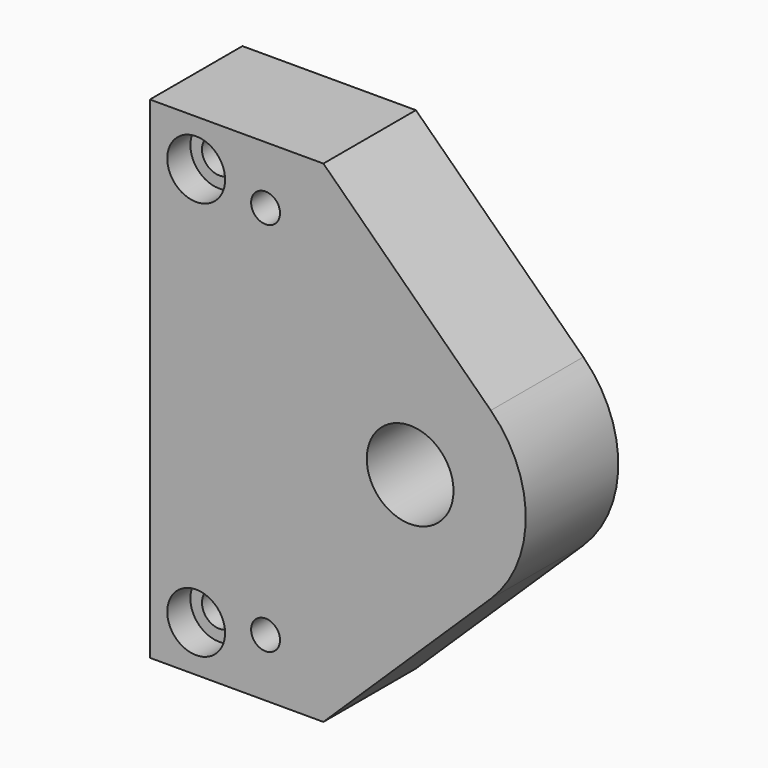
from build123d import *

# Parameters (mm, degrees)
F0_R           = 7.5
F1_DEPTH       = 20
F2_R           = 2.5
F3_DEPTH       = 20
F5_D           = 6
F5_DEPTH       = 20
F5_CBORE_D     = 10
F5_CBORE_DEPTH = 5
F5_TIP         = 1.8025818571


# Not quite as in the source:
# - a pattern or mirror of a feature is missing from the dataset's text; its kind, count and spacing are read off the source's solid


with BuildPart() as f1:
    # F0 (on Front) → F1 (new body)
    with BuildSketch(Plane.XZ):
        with BuildLine():
            Line((0, 42.5), (-30, 42.5))
            Line((-30, 42.5), (-30, -42.5))
            Line((-30, -42.5), (0, -42.5))
            Line((0, -42.5), (28.9472864716, -14.3343364017))
            ThreePointArc((28.9472864716, -14.3343364017), (35, 0), (28.9472864716, 14.3343364017))
            Line((28.9472864716, 14.3343364017), (0, 42.5))
        make_face()
        with Locations((15, 0)):
            Circle(F0_R, mode=Mode.SUBTRACT)
    extrude(amount=F1_DEPTH)

    # F2 (on face) → F3 (cut, through all)
    with BuildSketch(Plane.XZ.offset(20)):
        with Locations((-10, 32.5)):
            Circle(F2_R)
        with Locations((-10, -32.5)):
            Circle(F2_R)
    extrude(amount=-F3_DEPTH, mode=Mode.SUBTRACT)

    # F5
    with Locations(Plane.XZ.offset(20)):
        with Locations((-22, 34.5)):
            f5 = CounterBoreHole(F5_D / 2, F5_CBORE_D / 2, F5_CBORE_DEPTH, depth=F5_DEPTH)
            with Locations((0, 0, -(F5_DEPTH + F5_TIP / 2))):  # 118° drill point
                Cone(0, F5_D / 2, F5_TIP, mode=Mode.SUBTRACT)

    # F5_copies: F5 across plane
    add(f5.mirror(Plane(origin=(0, 0, 0), x_dir=(-1, 0, 0), z_dir=(0, 0, -1))), mode=Mode.SUBTRACT)


solid = f1.part
